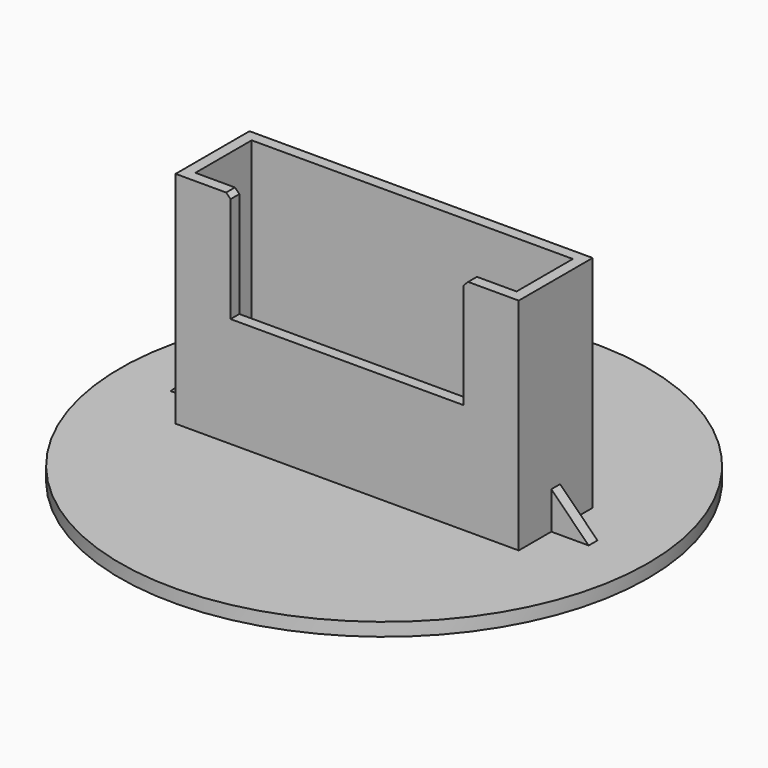
from build123d import *

# Parameters (mm, degrees)
F0_R         = 60
F0_W         = 8.5
F0_H         = 2.5
F0_W_2       = 2.5
F0_H_2       = 8.5
F2_DEPTH     = 3
F3_DEPTH     = 50
F4_T         = -2.5
F5_DEPTH     = 10
F6_T4_DEPTH  = 53.9336597593
F6_T10_DEPTH = 53.9336597593
F6_T16_DEPTH = 53.9336597593
F6_T22_DEPTH = 53.9336597593
F6_T28_DEPTH = 53.9336597593
F1_W         = 53
F1_H         = 50
F7_DEPTH     = 25
F8_SIZE      = 1


# Not quite as in the source:
# - a fillet or chamfer that OpenCascade refuses, or shapes differently, is made with other operations: its cross-section is extruded or revolved along the edge and cut away or added


with BuildPart() as f2:
    # F0 (on Top) → F2 (new body)
    with BuildSketch(Plane.XY):
        Circle(F0_R)
        Polygon((20, 10.5), (39, 10.5), (39, 1.25), (47.5, 1.25), (47.5, -1.25), (39, -1.25), (39, -10.5), (-39, -10.5), (-39, -1.25), (-47.5, -1.25), (-47.5, 1.25), (-39, 1.25), (-39, 10.5), (-20, 10.5), (-20, 19), (-17.5, 19), (-17.5, 10.5), (-1.25, 10.5), (-1.25, 19), (1.25, 19), (1.25, 10.5), (17.5, 10.5), (17.5, 19), (20, 19), align=None, mode=Mode.SUBTRACT)
        Polygon((39, 1.25), (39, 10.5), (20, 10.5), (17.5, 10.5), (1.25, 10.5), (-1.25, 10.5), (-17.5, 10.5), (-20, 10.5), (-39, 10.5), (-39, 1.25), (-39, -1.25), (-39, -10.5), (39, -10.5), (39, -1.25), align=None)
        with Locations((-43.25, 0)):
            Rectangle(F0_W, F0_H)
        with Locations((-18.75, 14.75)):
            Rectangle(F0_W_2, F0_H_2)
        with Locations((0, 14.75)):
            Rectangle(F0_W_2, F0_H_2)
        with Locations((18.75, 14.75)):
            Rectangle(F0_W_2, F0_H_2)
        with Locations((43.25, 0)):
            Rectangle(F0_W, F0_H)
    extrude(amount=-F2_DEPTH)

    # F0 (on Top) → F3 (join)
    with BuildSketch(Plane.XY):
        Polygon((39, 1.25), (39, 10.5), (20, 10.5), (17.5, 10.5), (1.25, 10.5), (-1.25, 10.5), (-17.5, 10.5), (-20, 10.5), (-39, 10.5), (-39, 1.25), (-39, -1.25), (-39, -10.5), (39, -10.5), (39, -1.25), align=None)
    extrude(amount=F3_DEPTH)

    # F4
    f4_openings = [f2.faces().sort_by_distance(p)[0] for p in [
        (0, 0, 50),
    ]]
    offset(amount=F4_T, openings=f4_openings, kind=Kind.INTERSECTION)

    # F0 (on Top) → F5 (join)
    with BuildSketch(Plane.XY):
        with Locations((18.75, 14.75)):
            Rectangle(F0_W_2, F0_H_2)
        with Locations((43.25, 0)):
            Rectangle(F0_W, F0_H)
        with Locations((0, 14.75)):
            Rectangle(F0_W_2, F0_H_2)
        with Locations((-18.75, 14.75)):
            Rectangle(F0_W_2, F0_H_2)
        with Locations((-43.25, 0)):
            Rectangle(F0_W, F0_H)
    extrude(amount=F5_DEPTH)

    # F6: chamfer of 10 on 5 edges, made by hand


with BuildPart() as f6_tool2:
    # F6_s3 → F6_t4 (new body)
    with BuildSketch(Plane.XZ.offset(26.9668298797)):
        Polygon((47.5, 0), (37.5, 10), (47.5, 10), align=None)
    extrude(amount=-F6_T4_DEPTH)

    split(bisect_by=Plane.XY, keep=Keep.TOP)

    split(bisect_by=Plane.YZ.offset(39), keep=Keep.TOP)


with BuildPart() as f2_1:
    add(f2.part)

    # F6_t1: cut F6_tool2
    add(f6_tool2.part, mode=Mode.SUBTRACT)


with BuildPart() as f6_tool8:
    # F6_s9 → F6_t10 (new body)
    with BuildSketch(Plane.YZ.offset(45.7168298797)):
        Polygon((19, 0), (9, 10), (19, 10), align=None)
    extrude(amount=-F6_T10_DEPTH)

    split(bisect_by=Plane.XY, keep=Keep.TOP)

    split(bisect_by=Plane.XZ.offset(-10.5), keep=Keep.BOTTOM)


with BuildPart() as f2_2:
    add(f2_1.part)

    # F6_t7: cut F6_tool8
    add(f6_tool8.part, mode=Mode.SUBTRACT)


with BuildPart() as f6_tool14:
    # F6_s15 → F6_t16 (new body)
    with BuildSketch(Plane.YZ.offset(26.9668298797)):
        Polygon((19, 0), (9, 10), (19, 10), align=None)
    extrude(amount=-F6_T16_DEPTH)

    split(bisect_by=Plane.XY, keep=Keep.TOP)

    split(bisect_by=Plane.XZ.offset(-10.5), keep=Keep.BOTTOM)


with BuildPart() as f2_3:
    add(f2_2.part)

    # F6_t13: cut F6_tool14
    add(f6_tool14.part, mode=Mode.SUBTRACT)


with BuildPart() as f6_tool20:
    # F6_s21 → F6_t22 (new body)
    with BuildSketch(Plane.YZ.offset(8.2168298797)):
        Polygon((19, 0), (9, 10), (19, 10), align=None)
    extrude(amount=-F6_T22_DEPTH)

    split(bisect_by=Plane.XY, keep=Keep.TOP)

    split(bisect_by=Plane.XZ.offset(-10.5), keep=Keep.BOTTOM)


with BuildPart() as f2_4:
    add(f2_3.part)

    # F6_t19: cut F6_tool20
    add(f6_tool20.part, mode=Mode.SUBTRACT)


with BuildPart() as f6_tool26:
    # F6_s27 → F6_t28 (new body)
    with BuildSketch(Plane.XZ.offset(-26.9668298797)):
        Polygon((-47.5, 0), (-37.5, 10), (-47.5, 10), align=None)
    extrude(amount=F6_T28_DEPTH)

    split(bisect_by=Plane.XY, keep=Keep.TOP)

    split(bisect_by=Plane.YZ.offset(-39), keep=Keep.BOTTOM)


with BuildPart() as f2_5:
    add(f2_4.part)

    # F6_t25: cut F6_tool26
    add(f6_tool26.part, mode=Mode.SUBTRACT)

    # F1 (on Front) → F7 (cut)
    with BuildSketch(Plane.XZ):
        with Locations((0, 50)):
            Rectangle(F1_W, F1_H)
    extrude(amount=F7_DEPTH, mode=Mode.SUBTRACT)

    # F8
    f8_edges = [f2_5.edges().sort_by_distance(p)[0] for p in [
        (-26.5, -9.25, 50),
        (26.5, -9.25, 50),
    ]]
    chamfer(f8_edges, length=F8_SIZE)


solid = f2_5.part
